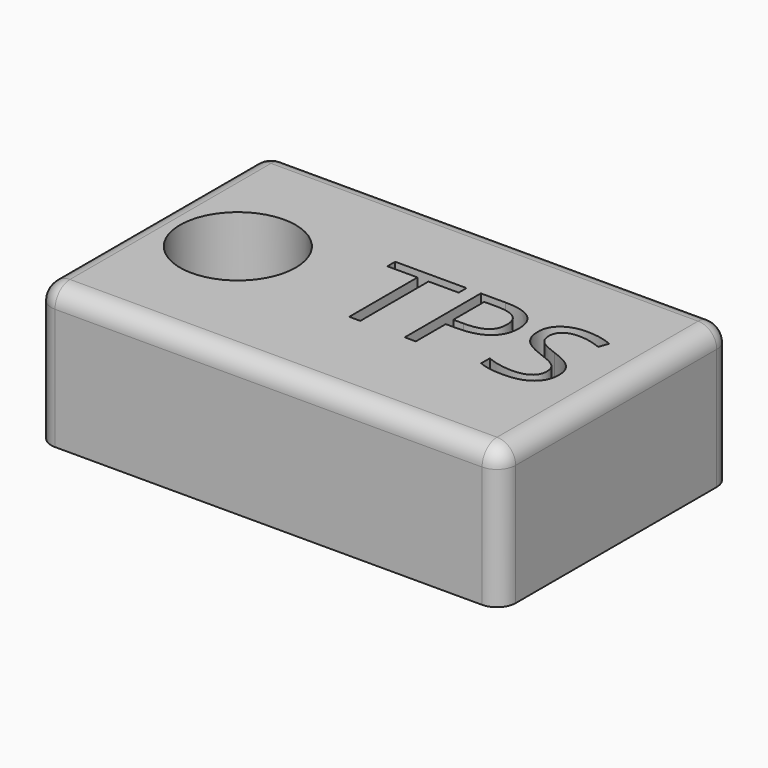
from build123d import *

# Parameters (mm, degrees)
F0_W         = 126.3902243227
F0_H         = 78.5530209541
F1_DEPTH     = 38.1
F2_TEXT_SIZE = 36.2655704117
F3_DEPTH     = 25.4
F4_R         = 5.08
F5_R         = 5.08
F6_R         = 5.08
F7_R         = 5.08
F8_R         = 15.7405872869
F9_DEPTH     = 27.94


# Not quite as in the source:
# - Text() gives the source's letters only with a copy of the font that has no kerning and outlines rounded to 1/6400 em; it was checked with that copy


with BuildPart() as f1:
    # F0 (on Top) → F1 (new body)
    with BuildSketch(Plane.XY):
        with Locations((-52.8699271381, 0)):
            Rectangle(F0_W, F0_H)
    extrude(amount=F1_DEPTH)

    # F2 (on face) → F3 (cut)
    with BuildSketch(Plane.XY.offset(38.1)):
        with Locations((-62.4164465757, -10.540464893)):
            Text('TPS', F2_TEXT_SIZE, font='Open Sans', text_align=(TextAlign.LEFT, TextAlign.BOTTOM))
    extrude(amount=-F3_DEPTH, mode=Mode.SUBTRACT)

    # F4
    f4_edges = [f1.edges().sort_by_distance(p)[0] for p in [
        (-116.065039, 0, 38.1),
    ]]
    fillet(f4_edges, radius=F4_R)

    # F5
    f5_edges = [f1.edges().sort_by_distance(p)[0] for p in [
        (-50.329927, -39.27651, 38.1),
    ]]
    fillet(f5_edges, radius=F5_R)

    # F6
    f6_edges = [f1.edges().sort_by_distance(p)[0] for p in [
        (10.325185, 2.54, 38.1),
    ]]
    fillet(f6_edges, radius=F6_R)

    # F7
    f7_edges = [f1.edges().sort_by_distance(p)[0] for p in [
        (-52.869927, 39.27651, 38.1),
    ]]
    fillet(f7_edges, radius=F7_R)

    # F8 (on face) → F9 (cut)
    with BuildSketch(Plane.XY.offset(38.1)):
        with Locations((-92.648178339, 0)):
            Circle(F8_R)
    extrude(amount=-F9_DEPTH, mode=Mode.SUBTRACT)


solid = f1.part
